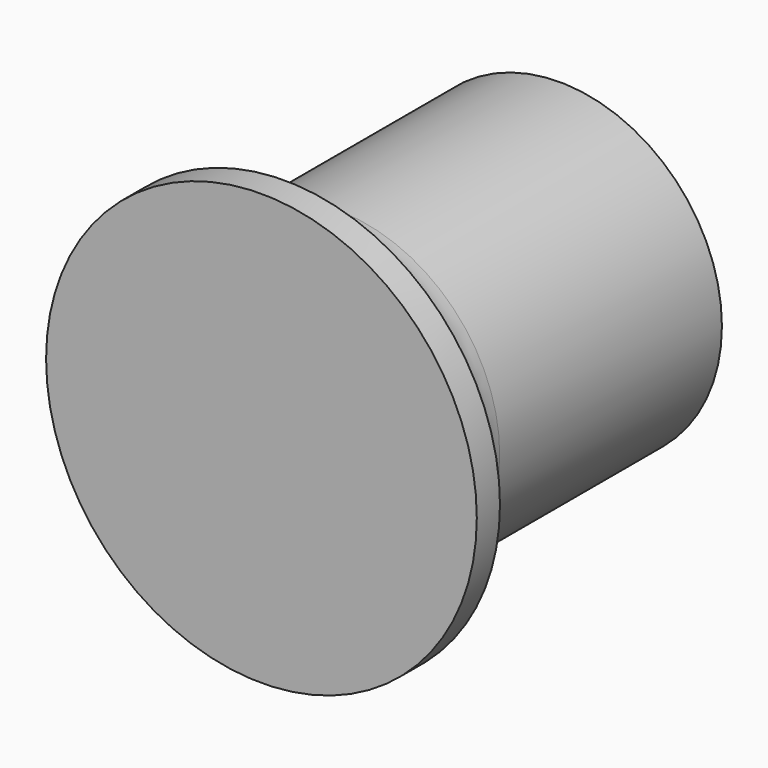
from build123d import *

# Parameters (mm, degrees)
F0_R     = 11.15
F1_DEPTH = 19.3
F3_START = -1.5
F2_R     = 11.15
F2_R_2   = 8.4
F3_DEPTH = 17.8


# Not quite as in the source:
# - a fillet or chamfer that OpenCascade refuses, or shapes differently, is made with other operations: its cross-section is extruded or revolved along the edge and cut away or added


with BuildPart() as f1:
    # F0 (on Front) → F1 (new body)
    with BuildSketch(Plane.XZ):
        Circle(F0_R)
    extrude(amount=F1_DEPTH)

    # F2 (on face) → F3 (cut)
    with BuildSketch(Plane.XZ.offset(19.3).offset(F3_START)):
        Circle(F2_R)
        Circle(F2_R_2, mode=Mode.SUBTRACT)
    extrude(amount=-F3_DEPTH, mode=Mode.SUBTRACT)

    # F4: fillet of radius 3.5 on 1 edges, made by hand

    # F4_s1 → F4_t2 (revolve)
    with BuildSketch(Plane.XY):
        with BuildLine():
            ThreePointArc((11.15, -17.8), (9.1728219713, -16.5750425141), (8.4, -14.3813014172))
            Line((8.4, -14.3813014172), (8.4, -17.8))
            Line((8.4, -17.8), (11.15, -17.8))
        make_face()
    revolve(axis=Axis((0, -17.8, 0), (0, -1, 0)))


solid = f1.part
